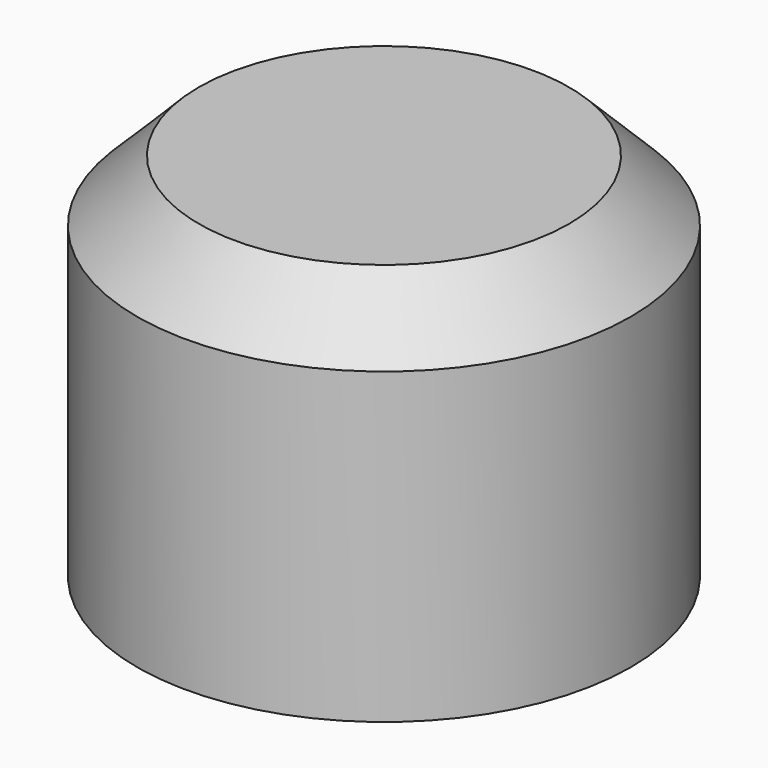
from build123d import *

# Parameters (mm, degrees)
F0_R     = 12.7
F1_DEPTH = 19.05
F2_SIZE  = 3.175
F3_T     = -3.175
F4_SIZE  = 3.17499


# Not quite as in the source:
# - a fillet or chamfer is up to 0.001 mm smaller than in the source, because OpenCascade refuses the exact size


with BuildPart() as f1:
    # F0 (on Top) → F1 (new body)
    with BuildSketch(Plane.XY):
        Circle(F0_R)
    extrude(amount=F1_DEPTH)

    # F2
    f2_edges = [f1.edges().sort_by_distance(p)[0] for p in [
        (-12.7, 0, 19.05),
    ]]
    chamfer(f2_edges, length=F2_SIZE)

    # F3
    f3_openings = [f1.faces().sort_by_distance(p)[0] for p in [
        (0, 0, 0),
    ]]
    offset(amount=F3_T, openings=f3_openings)

    # F4 (size 3.175 in the source; OpenCascade refuses exactly that, so slightly less here)
    f4_edges = [f1.edges().sort_by_distance(p)[0] for p in [
        (-9.525, 0, 0),
    ]]
    chamfer(f4_edges, length=F4_SIZE)


solid = f1.part
